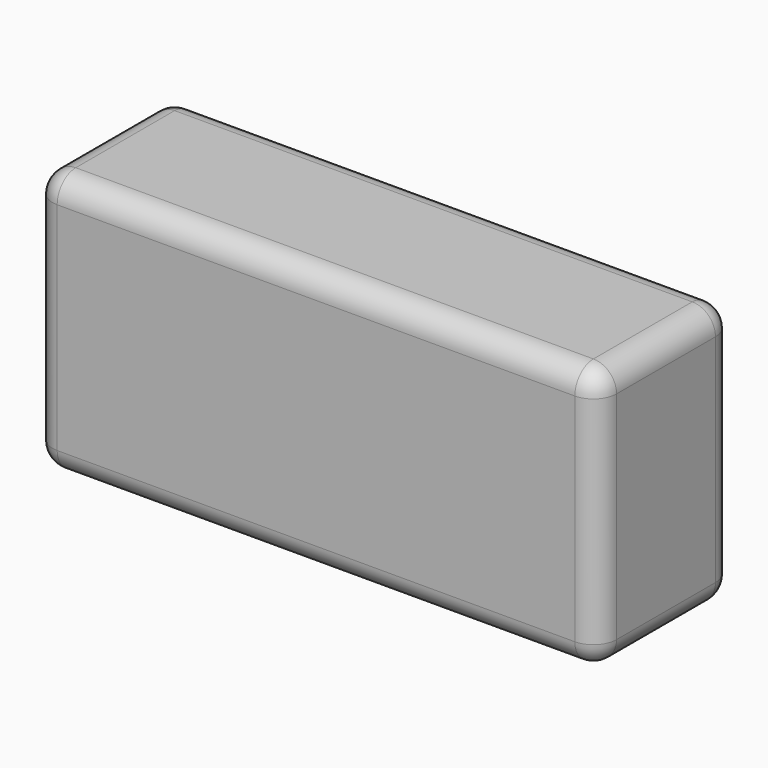
from build123d import *

# Parameters (mm, degrees)
F1_DEPTH = 34
F2_R     = 3


with BuildPart() as f1:
    # F0 (on Top) → F1 (new body)
    with BuildSketch(Plane.XY):
        with BuildLine():
            Line((33.5, 11), (-33.5, 11))
            ThreePointArc((-33.5, 11), (-35.6213203436, 10.1213203436), (-36.5, 8))
            Line((-36.5, 8), (-36.5, -8))
            ThreePointArc((-36.5, -8), (-35.6213203436, -10.1213203436), (-33.5, -11))
            Line((-33.5, -11), (33.5, -11))
            ThreePointArc((33.5, -11), (35.6213203436, -10.1213203436), (36.5, -8))
            Line((36.5, -8), (36.5, 8))
            ThreePointArc((36.5, 8), (35.6213203436, 10.1213203436), (33.5, 11))
        make_face()
    extrude(amount=F1_DEPTH)

    # F2
    f2_edges = [f1.edges().sort_by_distance(p)[0] for p in [
        (36.5, 0, 0),
        (35.62132, 10.12132, 0),
        (0, 11, 0),
        (-35.62132, 10.12132, 0),
        (-36.5, 0, 0),
        (-35.62132, -10.12132, 0),
        (0, -11, 0),
        (35.62132, -10.12132, 0),
        (36.5, 0, 34),
        (35.62132, 10.12132, 34),
        (0, 11, 34),
        (-35.62132, 10.12132, 34),
        (-36.5, 0, 34),
        (-35.62132, -10.12132, 34),
        (0, -11, 34),
        (35.62132, -10.12132, 34),
    ]]
    fillet(f2_edges, radius=F2_R)


solid = f1.part
